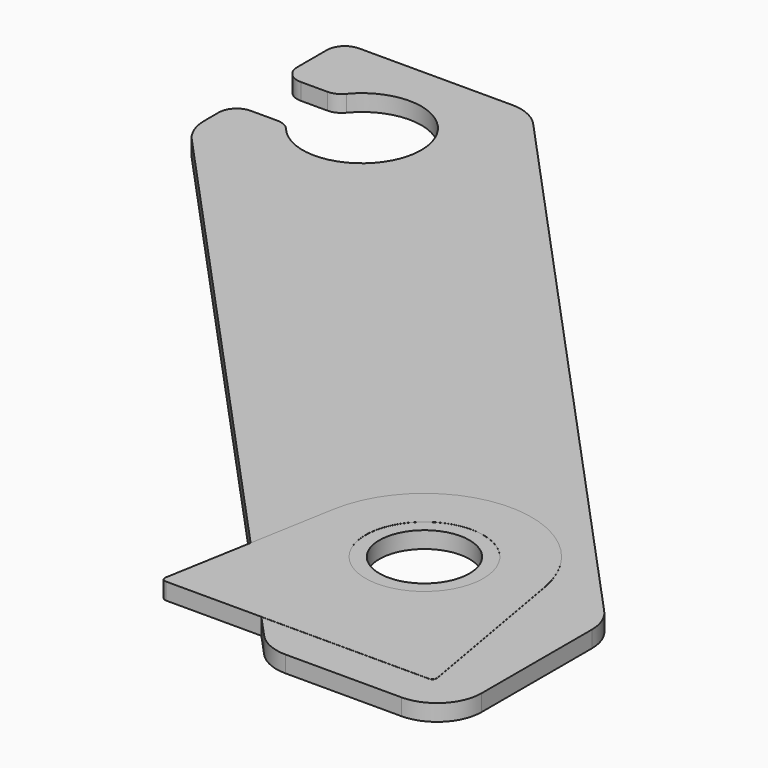
from build123d import *

# Parameters (mm, degrees)
F0_R     = 8.382
F1_DEPTH = 2.38125
F2_R     = 0.635
F3_R     = 6.4135
F4_DEPTH = 2.3622
F5_R     = 6.35
F6_R     = 2.54


# Not quite as in the source:
# - a feature names something its author has since deleted; it is built from what else it names


with BuildPart() as f1:
    # F0 (on Top) → F1 (new body)
    with BuildSketch(Plane.XY):
        with BuildLine():
            ThreePointArc((-15.24, 0), (0, -15.24), (15.24, 0))
            ThreePointArc((15.24, 0), (15.1820071989, 1.3282535195), (15.0084701559, 2.6463982276))
            ThreePointArc((15.0084701559, 2.6463982276), (0, 15.24), (-15.0084701559, 2.6463982276))
            ThreePointArc((-15.0084701559, 2.6463982276), (-15.1820071989, 1.3282535195), (-15.24, 0))
        make_face()
        Circle(F0_R, mode=Mode.SUBTRACT)
        with BuildLine():
            ThreePointArc((15.0084701559, 2.6463982276), (15.1820071989, 1.3282535195), (15.24, 0))
            ThreePointArc((15.24, 0), (0, -15.24), (-15.24, 0))
            ThreePointArc((-15.24, 0), (-15.1820071989, 1.3282535195), (-15.0084701559, 2.6463982276))
            Line((-15.0084701559, 2.6463982276), (-19.4626723496, -22.6146376946))
            ThreePointArc((-19.4626723496, -22.6146376946), (0, -17.78), (19.4626723496, -22.6146376946))
            Line((19.4626723496, -22.6146376946), (15.0084701559, 2.6463982276))
        make_face()
        with BuildLine():
            Line((-19.4626723496, -22.6146376946), (19.4626723496, -22.6146376946))
            ThreePointArc((19.4626723496, -22.6146376946), (0, -17.78), (-19.4626723496, -22.6146376946))
        make_face()
    extrude(amount=F1_DEPTH)

    # F2
    f2_edges = [f1.edges().sort_by_distance(p)[0] for p in [
        (-19.462672, -22.614638, 1.190625),
        (19.462672, -22.614638, 1.190625),
    ]]
    fillet(f2_edges, radius=F2_R)


with BuildPart() as f4:
    # F3 (on Top) → F4 (new body)
    with BuildSketch(Plane.XY):
        with BuildLine():
            ThreePointArc((-77.0311172703, 80.645), (-61.4045, 76.2), (-77.0311172703, 71.755))
            Line((-77.0311172703, 71.755), (-84.6455, 71.755))
            Line((-84.6455, 71.755), (-84.6455, 64.1485879677))
            Line((-84.6455, 64.1485879677), (-0.1727526963, -28.0035))
            Line((-0.1727526963, -28.0035), (25.4635, -28.0035))
            Line((25.4635, -28.0035), (25.4635, 0.4135938505))
            Line((25.4635, 0.4135938505), (-57.5699139704, 90.9955))
            Line((-57.5699139704, 90.9955), (-84.6455, 90.9955))
            Line((-84.6455, 90.9955), (-84.6455, 80.645))
            Line((-84.6455, 80.645), (-77.0311172703, 80.645))
        make_face()
        Circle(F3_R, mode=Mode.SUBTRACT)
    extrude(amount=F4_DEPTH)

    # F5
    f5_edges = [f4.edges().sort_by_distance(p)[0] for p in [
        (-57.569914, 90.9955, 1.1811),
        (25.4635, 0.413594, 1.1811),
        (25.4635, -28.0035, 1.1811),
        (-0.172753, -28.0035, 1.1811),
        (-84.6455, 64.148588, 1.1811),
    ]]
    fillet(f5_edges, radius=F5_R)

    # F6
    f6_edges = [f4.edges().sort_by_distance(p)[0] for p in [
        (-84.6455, 80.645, 1.1811),
        (-84.6455, 71.755, 1.1811),
        (-84.6455, 90.9955, 1.1811),
        (-77.031117, 80.645, 1.1811),
        (-77.031117, 71.755, 1.1811),
    ]]
    fillet(f6_edges, radius=F6_R)


solid = Compound([f1.part, f4.part])
